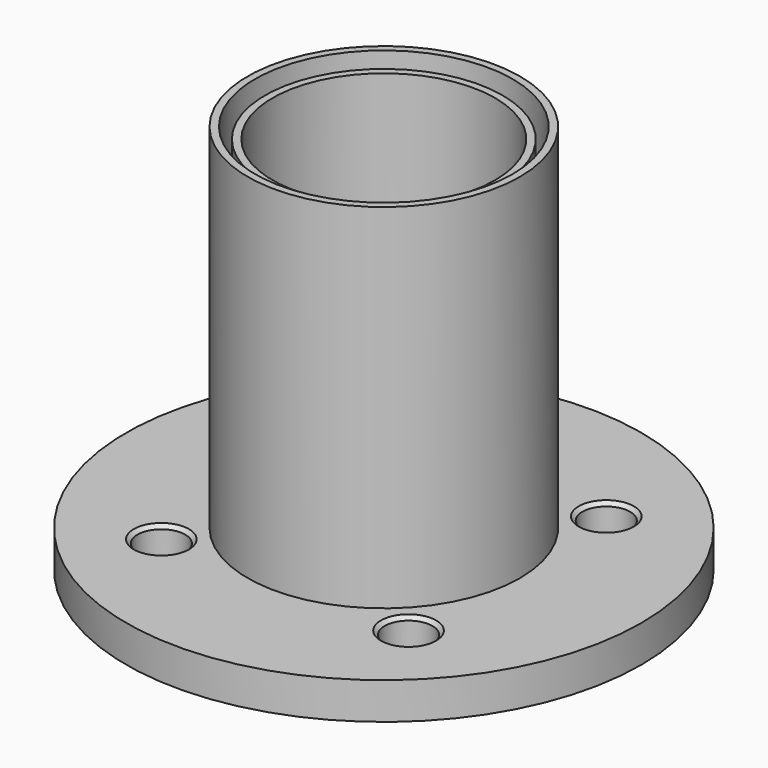
from build123d import *

# Parameters (mm, degrees)
F0_R      = 70
F0_R_2    = 6.5
F0_R_3    = 26.7709117697
F1_DEPTH  = 10
F2_R      = 30.15
F3_DEPTH  = 5
F4_R      = 31.25
F4_R_2    = 27.25
F5_DEPTH  = 25
F6_SIZE   = 1
F7_R      = 32.25
F7_R_2    = 30.25
F8_DEPTH  = 5
F9_R      = 37
F9_R_2    = 35
F10_DEPTH = 5
F11_R     = 32.25
F11_R_2   = 30.25
F12_DEPTH = 98
F13_R     = 37
F13_R_2   = 35
F14_DEPTH = 101
F15_R     = 32.25
F15_R_2   = 30.25
F16_DEPTH = 1.5


with BuildPart() as f1:
    # F0 (on Top) → F1 (new body)
    with BuildSketch(Plane.XY):
        Circle(F0_R)
        with Locations((-33.5875721064, -33.5875721064)):
            Circle(F0_R_2, mode=Mode.SUBTRACT)
        with Locations((33.5875721064, -33.5875721064)):
            Circle(F0_R_2, mode=Mode.SUBTRACT)
        with Locations((-33.5875721064, 33.5875721064)):
            Circle(F0_R_2, mode=Mode.SUBTRACT)
        Circle(F0_R_3, mode=Mode.SUBTRACT)
        with Locations((33.5875721064, 33.5875721064)):
            Circle(F0_R_2, mode=Mode.SUBTRACT)
    extrude(amount=F1_DEPTH)

    # F2 (on face) → F3 (cut)
    with BuildSketch(Plane(origin=(0, 0, 0), x_dir=(1, 0, 0), z_dir=(0, 0, -1))):
        Circle(F2_R)
    extrude(amount=-F3_DEPTH, mode=Mode.SUBTRACT)

    # F4 (on face) → F5 (join)
    with BuildSketch(Plane(origin=(0, 0, 5), x_dir=(1, 0, 0), z_dir=(0, 0, -1))):
        Circle(F4_R)
        Circle(F4_R_2, mode=Mode.SUBTRACT)
    extrude(amount=F5_DEPTH)

    # F6
    f6_edges = [f1.edges().sort_by_distance(p)[0] for p in [
        (-40.087572, 33.587572, 0),
        (27.087572, 33.587572, 0),
        (27.087572, -33.587572, 0),
        (-40.087572, -33.587572, 0),
        (27.087572, 33.587572, 10),
        (27.087572, -33.587572, 10),
        (-40.087572, -33.587572, 10),
        (-40.087572, 33.587572, 10),
    ]]
    chamfer(f6_edges, length=F6_SIZE)

    # F7 (on face) → F8 (cut)
    with BuildSketch(Plane.XY.offset(10)):
        Circle(F7_R)
        Circle(F7_R_2, mode=Mode.SUBTRACT)
    extrude(amount=-F8_DEPTH, mode=Mode.SUBTRACT)

    # F9 (on face) → F10 (cut)
    with BuildSketch(Plane.XY.offset(10)):
        Circle(F9_R)
        Circle(F9_R_2, mode=Mode.SUBTRACT)
    extrude(amount=-F10_DEPTH, mode=Mode.SUBTRACT)


with BuildPart() as f12:
    # F11 (on face) → F12 (new body)
    with BuildSketch(Plane.XY.offset(5)):
        Circle(F11_R)
        Circle(F11_R_2, mode=Mode.SUBTRACT)
    extrude(amount=F12_DEPTH)


with BuildPart() as f14:
    # F13 (on face) → F14 (new body)
    with BuildSketch(Plane.XY.offset(5)):
        Circle(F13_R)
        Circle(F13_R_2, mode=Mode.SUBTRACT)
    extrude(amount=F14_DEPTH)


with BuildPart() as f16:
    # F15 (on face) → F16 (new body)
    with BuildSketch(Plane.XY.offset(5)):
        Circle(F15_R)
        Circle(F15_R_2, mode=Mode.SUBTRACT)
    extrude(amount=F16_DEPTH)


solid = Compound([f1.part, f12.part, f14.part, f16.part])
